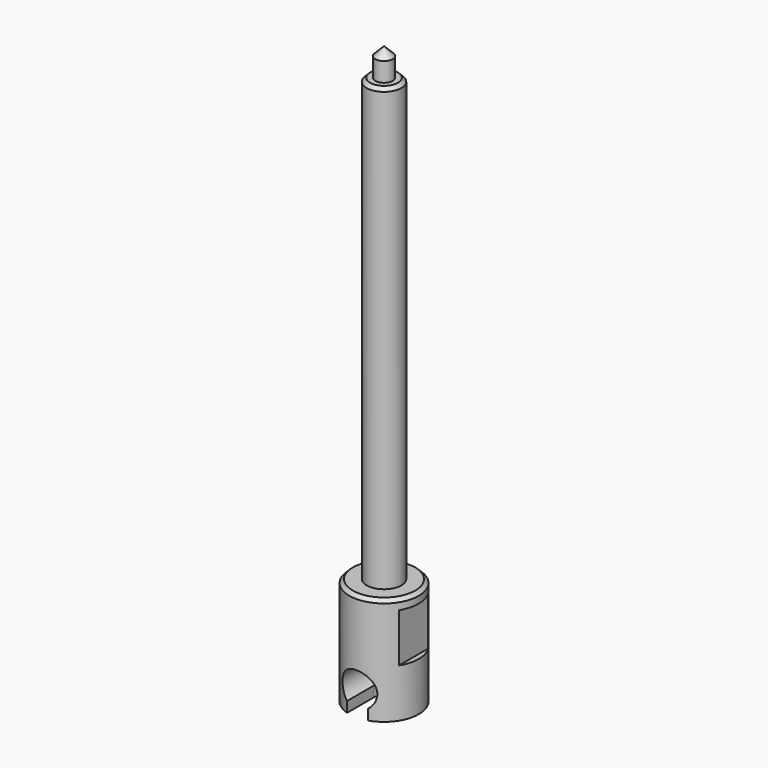
from build123d import *

# Parameters (mm, degrees)
F0_R      = 5
F1_DEPTH  = 127
F2_R      = 2.5
F3_DEPTH  = 8
F4_SIZE   = 2.5
F5_SIZE   = 1
F6_R      = 10
F6_R_2    = 5
F7_DEPTH  = 31
F9_R      = 5
F10_DEPTH = 15
F12_DEPTH = 8
F13_SIZE  = 1
F15_W     = 11.5
F15_H     = 14
F16_DEPTH = 1.5


# Not quite as in the source:
# - a pattern or mirror of a feature is missing from the dataset's text; its kind, count and spacing are read off the source's solid


with BuildPart() as f1:
    # F0 (on Top) → F1 (new body)
    with BuildSketch(Plane.XY):
        Circle(F0_R)
    extrude(amount=F1_DEPTH)

    # F2 (on face) → F3 (join)
    with BuildSketch(Plane.XY.offset(127)):
        Circle(F2_R)
    extrude(amount=F3_DEPTH)

    # F4
    f4_edges = [f1.edges().sort_by_distance(p)[0] for p in [
        (-2.5, 0, 135),
    ]]
    chamfer(f4_edges, length=F4_SIZE)

    # F5
    f5_edges = [f1.edges().sort_by_distance(p)[0] for p in [
        (-5, 0, 127),
    ]]
    chamfer(f5_edges, length=F5_SIZE)

    # F6 (on face) → F7 (join)
    with BuildSketch(Plane(origin=(0, 0, 0), x_dir=(1, 0, 0), z_dir=(0, 0, -1))):
        Circle(F6_R)
        Circle(F6_R_2, mode=Mode.SUBTRACT)
        Circle(F6_R_2)
    extrude(amount=F7_DEPTH)

    # F9 (on offset) → F10 (cut)
    with BuildSketch(Plane.XZ.offset(10)):
        with Locations((0, -24)):
            Circle(F9_R)
    extrude(amount=-F10_DEPTH, mode=Mode.SUBTRACT)

    # F11 (on face) → F12 (cut)
    with BuildSketch(Plane(origin=(0, 0, -31), x_dir=(1, 0, 0), z_dir=(0, 0, -1))):
        with BuildLine():
            Line((-3, 9.5393920142), (-3, 0))
            ThreePointArc((-3, 0), (0, -3), (3, 0))
            Line((3, 0), (3, 9.5393920142))
            ThreePointArc((3, 9.5393920142), (0, 10), (-3, 9.5393920142))
        make_face()
    extrude(amount=-F12_DEPTH, mode=Mode.SUBTRACT)

    # F13
    f13_edges = [f1.edges().sort_by_distance(p)[0] for p in [
        (-10, 0, 0),
    ]]
    chamfer(f13_edges, length=F13_SIZE)

    # F15 (on offset) → F16 (cut)
    with BuildSketch(Plane.YZ.offset(10)):
        with Locations((0, -10)):
            Rectangle(F15_W, F15_H)
    f16 = extrude(amount=-F16_DEPTH, mode=Mode.SUBTRACT)

    # F16_copies: F16 across plane
    add(f16.mirror(Plane(origin=(0, 0, 0), x_dir=(0, 0, -1), z_dir=(-1, 0, 0))), mode=Mode.SUBTRACT)


solid = f1.part
